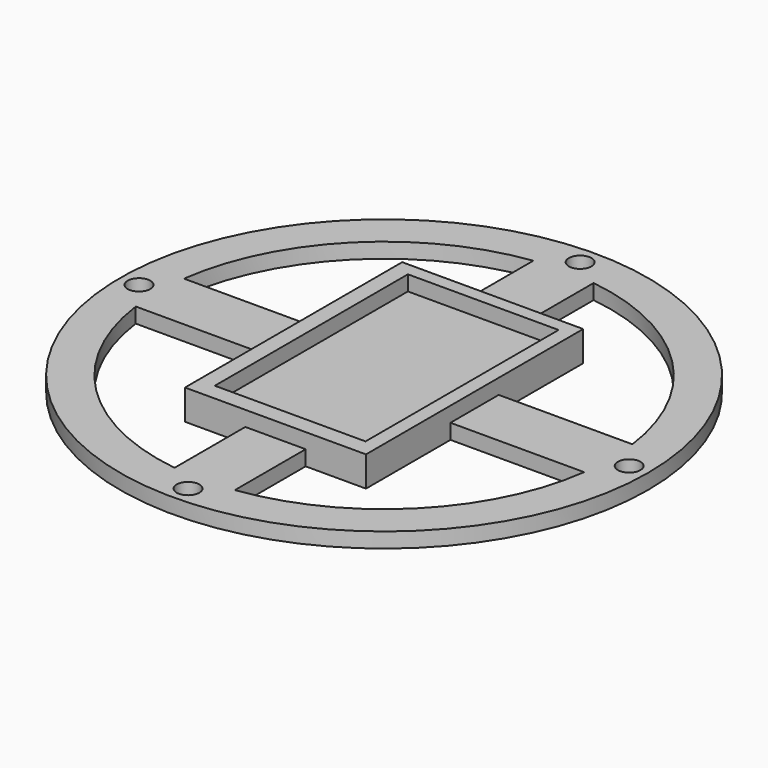
from build123d import *

# Parameters (mm, degrees)
F0_R     = 35
F0_R_2   = 1.5
F0_W     = 19.983293198
F0_H     = 32
F1_DEPTH = 2
F2_DEPTH = 4


# Not quite as in the source:
# - a feature names something its author has since deleted; it is built from what else it names


with BuildPart() as f1:
    # F0 (on Top) → F1 (new body)
    with BuildSketch(Plane.XY):
        Circle(F0_R)
        with Locations((0, -32.5)):
            Circle(F0_R_2, mode=Mode.SUBTRACT)
        with Locations((-32.5, 0)):
            Circle(F0_R_2, mode=Mode.SUBTRACT)
        with BuildLine():
            ThreePointArc((29.7321374946, 4), (29.9329594664, 2.0044793789), (30, 0))
            ThreePointArc((30, 0), (29.9329594664, -2.0044793789), (29.7321374946, -4))
            ThreePointArc((29.7321374946, -4), (21.2132034356, -21.2132034356), (4, -29.7321374946))
            ThreePointArc((4, -29.7321374946), (0, -30), (-4, -29.7321374946))
            ThreePointArc((-4, -29.7321374946), (-21.2132034356, -21.2132034356), (-29.7321374946, -4))
            ThreePointArc((-29.7321374946, -4), (-30, 0), (-29.7321374946, 4))
            ThreePointArc((-29.7321374946, 4), (-21.2132034356, 21.2132034356), (-4, 29.7321374946))
            ThreePointArc((-4, 29.7321374946), (0, 30), (4, 29.7321374946))
            ThreePointArc((4, 29.7321374946), (21.2132034356, 21.2132034356), (29.7321374946, 4))
        make_face(mode=Mode.SUBTRACT)
        with Locations((32.5, 0)):
            Circle(F0_R_2, mode=Mode.SUBTRACT)
        with Locations((0, 32.5)):
            Circle(F0_R_2, mode=Mode.SUBTRACT)
        with BuildLine():
            Line((4, 18), (4, 29.7321374946))
            ThreePointArc((4, 29.7321374946), (0, 30), (-4, 29.7321374946))
            Line((-4, 29.7321374946), (-4, 18))
            Line((-4, 18), (4, 18))
        make_face()
        with BuildLine():
            Line((-12, 4), (-29.7321374946, 4))
            ThreePointArc((-29.7321374946, 4), (-30, 0), (-29.7321374946, -4))
            Line((-29.7321374946, -4), (-12, -4))
            Line((-12, -4), (-12, 4))
        make_face()
        with BuildLine():
            ThreePointArc((-4, -29.7321374946), (0, -30), (4, -29.7321374946))
            Line((4, -29.7321374946), (4, -18))
            Line((4, -18), (-4, -18))
            Line((-4, -18), (-4, -29.7321374946))
        make_face()
        Polygon((12, -4), (12, 4), (12, 12.1005004627), (12, 18), (4, 18), (-4, 18), (-12, 18), (-12, 4), (-12, -4), (-12, -18), (-4, -18), (4, -18), (12, -18), (12, -5.151443038), align=None)
        with Locations((0.1530251862, 0.242334145)):
            Rectangle(F0_W, F0_H, mode=Mode.SUBTRACT)
        with Locations((0.1530251862, 0.242334145)):
            Rectangle(F0_W, F0_H)
        with BuildLine():
            ThreePointArc((29.7321374946, -4), (29.9329594664, -2.0044793789), (30, 0))
            ThreePointArc((30, 0), (29.9329594664, 2.0044793789), (29.7321374946, 4))
            Line((29.7321374946, 4), (12, 4))
            Line((12, 4), (12, -4))
            Line((12, -4), (29.7321374946, -4))
        make_face()
    extrude(amount=F1_DEPTH)

    # F0 (on Top) → F2 (join)
    with BuildSketch(Plane.XY):
        Polygon((12, -4), (12, 4), (12, 12.1005004627), (12, 18), (4, 18), (-4, 18), (-12, 18), (-12, 4), (-12, -4), (-12, -18), (-4, -18), (4, -18), (12, -18), (12, -5.151443038), align=None)
        with Locations((0.1530251862, 0.242334145)):
            Rectangle(F0_W, F0_H, mode=Mode.SUBTRACT)
    extrude(amount=F2_DEPTH)


solid = f1.part
